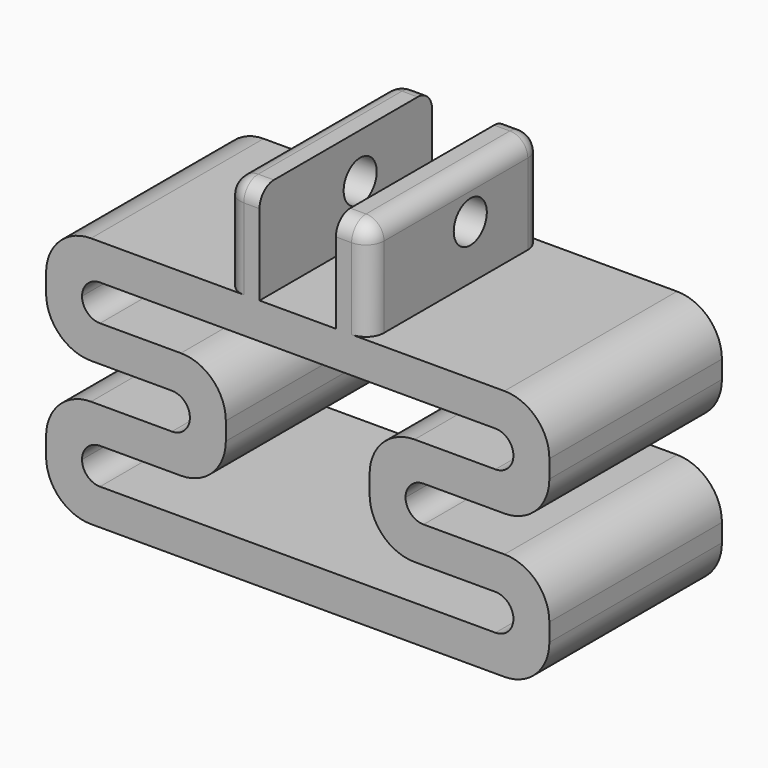
from build123d import *

# Parameters (mm, degrees)
F0_W     = 3.75
F0_H     = 11
F1_DEPTH = 24
F3_DEPTH = 24.001
F4_D     = 4.6
F5_R     = 1.99999
F6_R     = 5


# Not quite as in the source:
# - a fillet or chamfer is up to 0.001 mm smaller than in the source, because OpenCascade refuses the exact size


with BuildPart() as f1:
    # F0 (on Front) → F1 (new body)
    with BuildSketch(Plane.XZ):
        Polygon((0, 0), (-4.25, 0), (-8, 0), (-28, 0), (-28, -12), (-12, -12), (-12, -16), (-28, -16), (-28, -28), (0, -28), (0, -24), (-8, -24), (-24, -24), (-24, -20), (-8, -20), (-8, -11), (-8, -8), (-24, -8), (-24, -4), (-8, -4), (0, -4), align=None)
        Polygon((28, 0), (8, 0), (8, -4), (24, -4), (24, -8), (8, -8), (8, -11), (8, -20), (24, -20), (24, -24), (8, -24), (0, -24), (0, -28), (28, -28), (28, -16), (12, -16), (12, -12), (28, -12), align=None)
        Polygon((8, -4), (8, 0), (4.25, 0), (0, 0), (0, -4), align=None)
        with Locations((6.125, 5.5)):
            Rectangle(F0_W, F0_H)
        Polygon((4.25, 0), (4.25, 11), (-4.25, 11), (-4.25, 0), (0, 0), align=None)
        with Locations((-6.125, 5.5)):
            Rectangle(F0_W, F0_H)
    extrude(amount=F1_DEPTH)

    # F0 (on Front) → F3 (cut, through all)
    with BuildSketch(Plane.XZ):
        Polygon((4.25, 0), (4.25, 11), (-4.25, 11), (-4.25, 0), (0, 0), align=None)
    extrude(amount=F3_DEPTH, mode=Mode.SUBTRACT)

    # F4 (through all)
    with Locations(Plane.YZ.offset(8)):
        with Locations((-10, 6)):
            Hole(F4_D / 2)

    # F5 (radius 2 in the source; OpenCascade refuses exactly that, so slightly less here)
    f5_edges = [f1.edges().sort_by_distance(p)[0] for p in [
        (12, -12, -16),
        (-24, -12, -24),
        (-24, -12, -8),
        (12, -12, -12),
        (24, -12, -8),
        (24, -12, -24),
        (-12, -12, -12),
        (24, -12, -20),
        (24, -12, -4),
        (-24, -12, -20),
        (-24, -12, -4),
        (-12, -12, -16),
        (-8, -12, 11),
        (-6.125, -24, 11),
        (6.125, -24, 11),
        (8, -12, 11),
        (-8, 0, 5.5),
        (-8, -24, 5.5),
        (-6.125, 0, 11),
        (6.125, 0, 11),
        (8, 0, 5.5),
        (8, -24, 5.5),
    ]]
    fillet(f5_edges, radius=F5_R)

    # F6
    f6_edges = [f1.edges().sort_by_distance(p)[0] for p in [
        (-28, -12, -28),
        (-28, -12, -16),
        (-28, -12, -12),
        (-28, -12, 0),
        (8, -12, -8),
        (8, -12, -20),
        (-8, -12, -8),
        (-8, -12, -20),
        (28, -12, 0),
        (28, -12, -12),
        (28, -12, -16),
        (28, -12, -28),
    ]]
    fillet(f6_edges, radius=F6_R)


solid = f1.part
